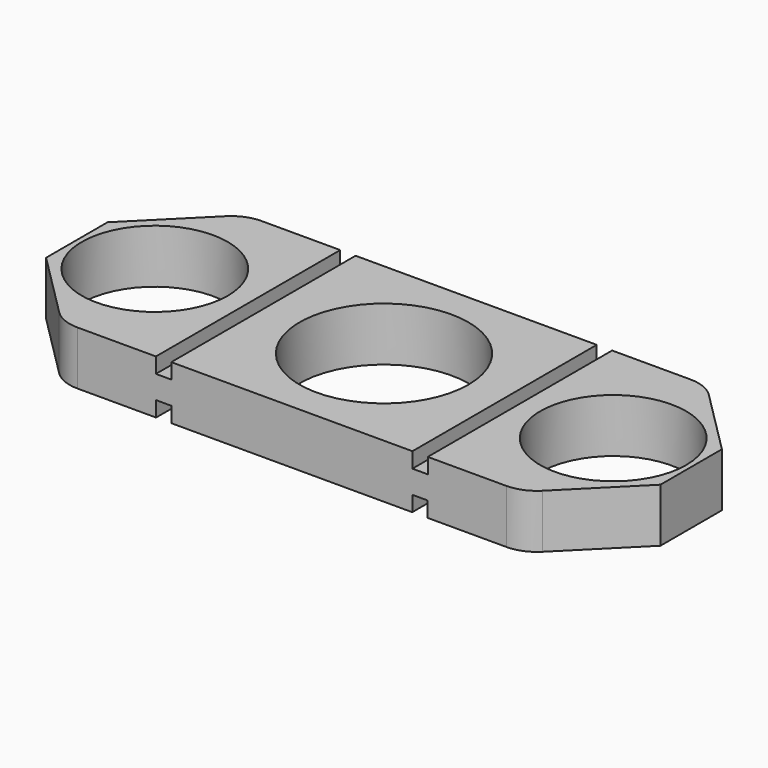
from build123d import *

# Parameters (mm, degrees)
F0_W      = 80
F0_H      = 30
F1_DEPTH  = 7
F2_R      = 11
F3_DEPTH  = 7.001
F4_SIZE   = 10
F5_R      = 5
F6_R      = 9.5
F7_DEPTH  = 7.001
F8_W      = 2
F8_H      = 30
F9_DEPTH  = 2
F10_W     = 2
F10_H     = 30
F11_DEPTH = 2


with BuildPart() as f1:
    # F0 (on Top) → F1 (new body)
    with BuildSketch(Plane.XY):
        Rectangle(F0_W, F0_H)
    extrude(amount=F1_DEPTH)

    # F2 (on face) → F3 (cut, through all)
    with BuildSketch(Plane.XY.offset(7)):
        Circle(F2_R)
    extrude(amount=-F3_DEPTH, mode=Mode.SUBTRACT)

    # F4
    f4_edges = [f1.edges().sort_by_distance(p)[0] for p in [
        (-40, 15, 3.5),
        (40, -15, 3.5),
        (40, 15, 3.5),
        (-40, -15, 3.5),
    ]]
    chamfer(f4_edges, length=F4_SIZE)

    # F5
    f5_edges = [f1.edges().sort_by_distance(p)[0] for p in [
        (-30, 15, 3.5),
        (-30, -15, 3.5),
        (30, -15, 3.5),
        (30, 15, 3.5),
    ]]
    fillet(f5_edges, radius=F5_R)

    # F6 (on face) → F7 (cut, through all)
    with BuildSketch(Plane.XY.offset(7)):
        with Locations((29.84234935, 0)):
            Circle(F6_R)
        with Locations((-29.84234935, 0)):
            Circle(F6_R)
    extrude(amount=-F7_DEPTH, mode=Mode.SUBTRACT)

    # F8 (on face) → F9 (cut)
    with BuildSketch(Plane.XY.offset(7)):
        with Locations((16.7006367594, 0)):
            Rectangle(F8_W, F8_H)
        with Locations((-16.7006367594, 0)):
            Rectangle(F8_W, F8_H)
    extrude(amount=-F9_DEPTH, mode=Mode.SUBTRACT)

    # F10 (on face) → F11 (cut)
    with BuildSketch(Plane(origin=(0, 0, 0), x_dir=(1, 0, 0), z_dir=(0, 0, -1))):
        with Locations((16.6785700023, 0)):
            Rectangle(F10_W, F10_H)
        with Locations((-16.6785700023, 0)):
            Rectangle(F10_W, F10_H)
    extrude(amount=-F11_DEPTH, mode=Mode.SUBTRACT)


solid = f1.part
